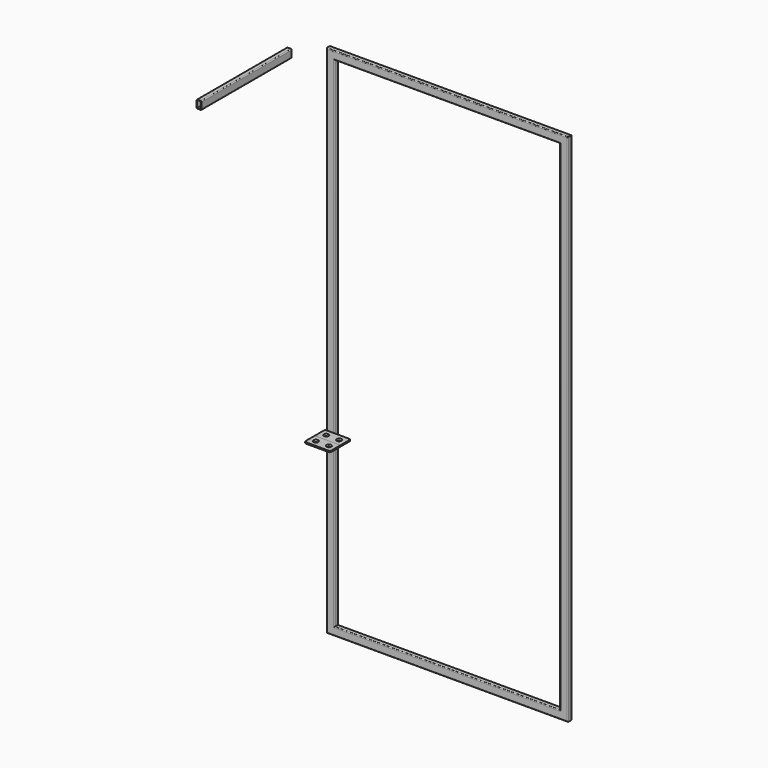
from build123d import *

# Parameters (mm, degrees)
F0_W     = 750
F0_H     = 1600
F0_W_2   = 700
F0_H_2   = 1550
F1_DEPTH = 15
F2_W     = 15
F2_H     = 25
F2_W_2   = 12
F2_H_2   = 22
F3_DEPTH = 350
F4_R     = 2.5
F5_DEPTH = 4
F8_R     = 2.5
F8_2_R   = 2.5
F9_R     = 2.5


# Not quite as in the source:
# - a fillet or chamfer that OpenCascade refuses, or shapes differently, is made with other operations: its cross-section is extruded or revolved along the edge and cut away or added


with BuildPart() as f1:
    # F0 (on Front) → F1 (new body)
    with BuildSketch(Plane.XZ):
        Rectangle(F0_W, F0_H)
        Rectangle(F0_W_2, F0_H_2, mode=Mode.SUBTRACT)
    extrude(amount=-F1_DEPTH)

    # F8
    f8_edges = [f1.edges().sort_by_distance(p)[0] for p in [
        (-350, 0, 0),
        (0, 0, 775),
        (350, 0, 0),
        (0, 15, -775),
        (0, 0, -775),
        (-350, 15, 0),
        (0, 15, 775),
    ]]
    fillet(f8_edges, radius=F8_R)

    # F9
    f9_edges = [f1.edges().sort_by_distance(p)[0] for p in [
        (-375, 15, 0),
        (-375, 0, 0),
        (0, 15, 800),
        (0, 0, 800),
        (375, 0, 0),
        (375, 15, 0),
        (0, 15, -800),
        (0, 0, -800),
    ]]
    fillet(f9_edges, radius=F9_R)


with BuildPart() as f3:
    # F2 (on face) → F3 (new body)
    with BuildSketch(Plane.XZ):
        with Locations((-490.5836057663, 749.3983626366)):
            Rectangle(F2_W, F2_H)
        with Locations((-490.5836057663, 749.3983626366)):
            Rectangle(F2_W_2, F2_H_2, mode=Mode.SUBTRACT)
    extrude(amount=F3_DEPTH)

    # F8#2
    f8_2_edges = [f3.edges().sort_by_distance(p)[0] for p in [
        (-483.083606, -175, 736.898363),
        (-498.083606, -175, 761.898363),
        (-483.083606, -175, 761.898363),
        (-498.083606, -175, 736.898363),
    ]]
    fillet(f8_2_edges, radius=F8_2_R)


with BuildPart() as f5:
    # F4 (on Top) → F5 (new body)
    with BuildSketch(Plane.XY):
        with BuildLine():
            Line((-5, -374.3908321857), (-75, -374.3908321857))
            ThreePointArc((-75, -374.3908321857), (-78.5355339059, -375.8552982798), (-80, -379.3908321857))
            Line((-80, -379.3908321857), (-80, -414.3908321857))
            Line((-80, -414.3908321857), (0, -414.3908321857))
            Line((0, -414.3908321857), (0, -379.3908321857))
            ThreePointArc((0, -379.3908321857), (-1.4644660941, -375.8552982798), (-5, -374.3908321857))
        make_face()
        with Locations((-60, -394.3908321857)):
            Circle(F4_R, mode=Mode.SUBTRACT)
        with Locations((-20, -394.3908321857)):
            Circle(F4_R, mode=Mode.SUBTRACT)
    extrude(amount=F5_DEPTH)

    # F6: chamfer of 5 on 2 edges, made by hand

    # F6_s1 → F6_t2 (revolve, cut)
    with BuildSketch(Plane.XZ.offset(394.3908321857)):
        Polygon((-17.5, -1), (-12.5, 4), (-17.5, 4), align=None)
    revolve(axis=Axis((-20, -394.3908321857, 4), (0, 0, 1)), mode=Mode.SUBTRACT)

    # F6_s3 → F6_t4 (revolve, cut)
    with BuildSketch(Plane.XZ.offset(394.3908321857)):
        Polygon((-57.5, -1), (-52.5, 4), (-57.5, 4), align=None)
    revolve(axis=Axis((-60, -394.3908321857, 4), (0, 0, 1)), mode=Mode.SUBTRACT)


with BuildPart() as f7_1:
    # F7: instance of F5
    add(f5.part.mirror(Plane(origin=(-40, -414.3908321857, 2), x_dir=(1, 0, 0), z_dir=(0, -1, 0))))


solid = Compound([f1.part, f3.part, f5.part, f7_1.part])
